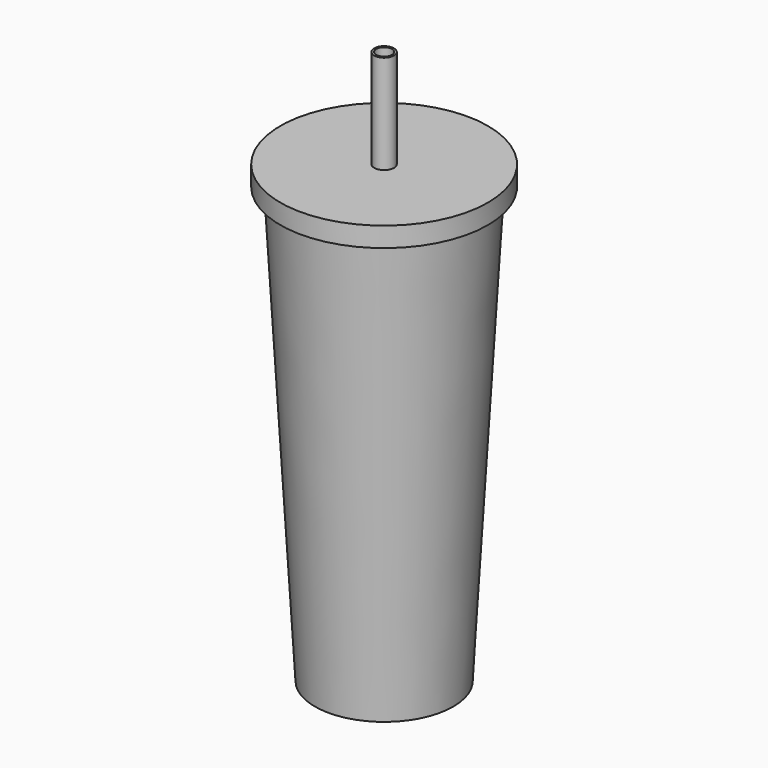
from build123d import *

# Parameters (mm, degrees)
F0_R     = 47.5
F2_R     = 35
F4_R     = 52.5
F4_R_2   = 47.5
F5_DEPTH = 10
F6_R     = 5
F6_R_2   = 4
F7_DEPTH = 50


with BuildPart() as f3:
    # F0 (on Top) → F3 section 0
    with BuildSketch(Plane.XY):
        Circle(F0_R)
    # F2 (on offset) → F3 section 1
    with BuildSketch(Plane.XY.offset(-220)):
        Circle(F2_R)
    loft()

    # F4 (on face) → F5 (join)
    with BuildSketch(Plane.XY):
        Circle(F4_R)
        Circle(F4_R_2, mode=Mode.SUBTRACT)
        Circle(F4_R_2)
    extrude(amount=F5_DEPTH)

    # F6 (on face) → F7 (join)
    with BuildSketch(Plane.XY.offset(10)):
        Circle(F6_R)
        Circle(F6_R_2, mode=Mode.SUBTRACT)
    extrude(amount=F7_DEPTH)


solid = f3.part
